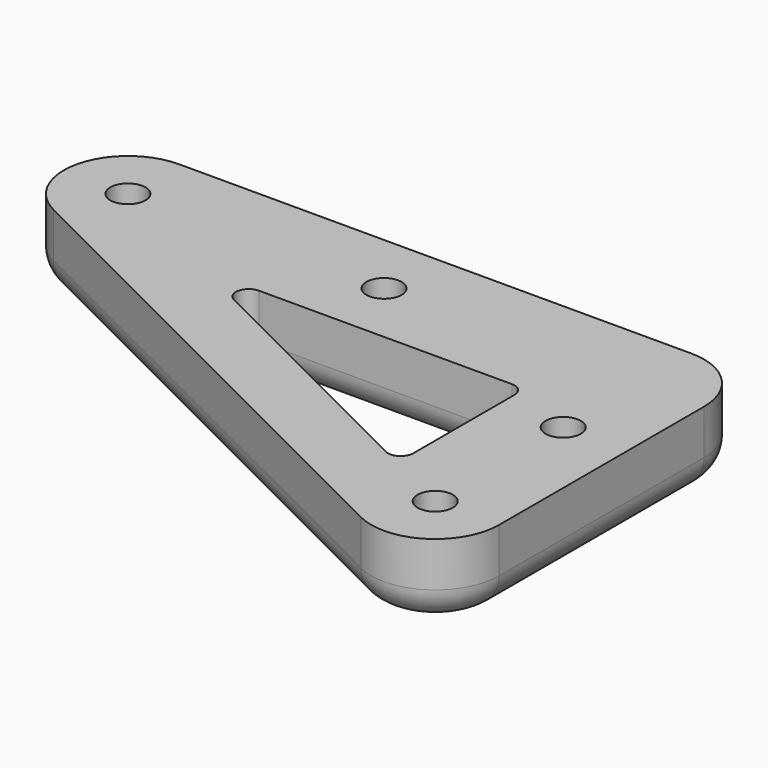
from build123d import *

# Parameters (mm, degrees)
F1_DEPTH       = 12
F2_D           = 5.5
F2_CBORE_D     = 9.75
F2_CBORE_DEPTH = 5
F3_R           = 4.99999


# Not quite as in the source:
# - a fillet or chamfer is up to 0.001 mm smaller than in the source, because OpenCascade refuses the exact size


with BuildPart() as f1:
    # F0 (on Top) → F1 (new body)
    with BuildSketch(Plane.XY):
        with BuildLine():
            ThreePointArc((-80, 10), (-89.7324898947, 2.2975292055), (-84.472135955, -8.94427191))
            Line((-84.472135955, -8.94427191), (-4.472135955, -48.94427191))
            ThreePointArc((-4.472135955, -48.94427191), (5.2573111212, -48.5065080835), (10, -40))
            Line((10, -40), (10, 0))
            ThreePointArc((10, 0), (7.0710678119, 7.0710678119), (0, 10))
            Line((0, 10), (-80, 10))
        make_face()
        with BuildLine():
            Line((-12.894427191, -33.5527864045), (-52.422291236, -13.788854382))
            ThreePointArc((-52.422291236, -13.788854382), (-53.4743620239, -11.5404941589), (-51.527864045, -10))
            Line((-51.527864045, -10), (-12, -10))
            ThreePointArc((-12, -10), (-10.5857864376, -10.5857864376), (-10, -12))
            Line((-10, -12), (-10, -31.7639320225))
            ThreePointArc((-10, -31.7639320225), (-10.9485377758, -33.4652336392), (-12.894427191, -33.5527864045))
        make_face(mode=Mode.SUBTRACT)
    extrude(amount=F1_DEPTH)

    # F2 (through all)
    with Locations(Plane(origin=(0, 0, 0), x_dir=(1, 0, 0), z_dir=(0, 0, -1))):
        with Locations((0, 40), (-40, 0), (-80, 0), (0, 15)):
            CounterBoreHole(F2_D / 2, F2_CBORE_D / 2, F2_CBORE_DEPTH)

    # F3 (radius 5 in the source; OpenCascade refuses exactly that, so slightly less here)
    f3_edges = [f1.edges().sort_by_distance(p)[0] for p in [
        (-40, 10, 0),
        (-31.763932, -10, 0),
    ]]
    fillet(f3_edges, radius=F3_R)


solid = f1.part
